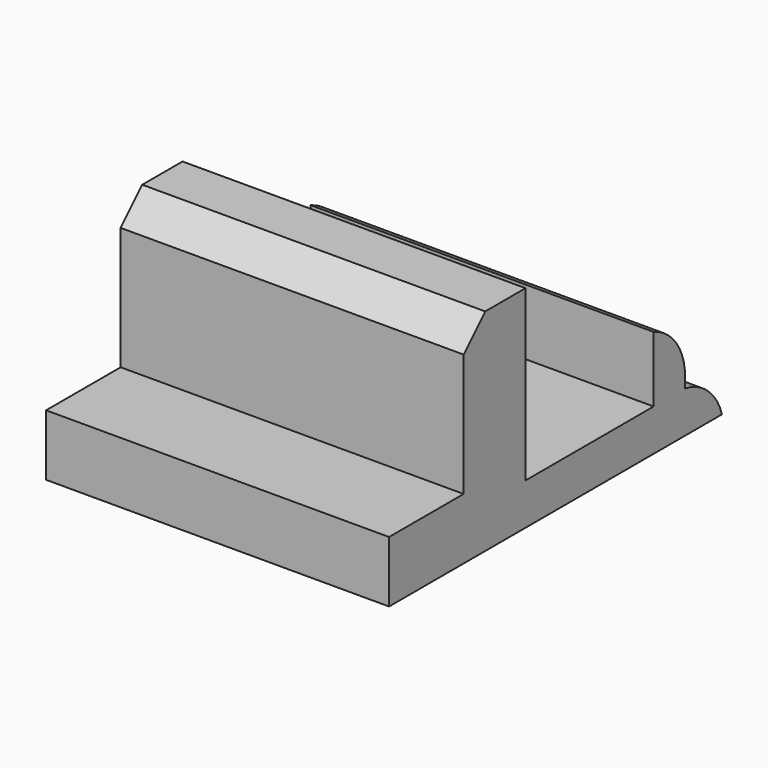
from build123d import *

# Parameters (mm, degrees)
F0_W        = 17.2521322966
F0_H        = 11.3339135423
F1_DEPTH    = 63.5
F2_T1_DEPTH = 116.9691747536
F2_T3_DEPTH = 114.7757874589
F3_SIZE     = 5


# Not quite as in the source:
# - a fillet or chamfer that OpenCascade refuses, or shapes differently, is made with other operations: its cross-section is extruded or revolved along the edge and cut away or added


with BuildPart() as f1:
    # F0 (on Right) → F1 (new body)
    with BuildSketch(Plane.YZ):
        Polygon((-28.8866702467, 39.0534885228), (-43.2048514485, 39.0534885228), (-43.2048514485, 11.3339135423), (-43.2048514485, 0), (16.9898695312, 0), (16.9898695312, 7.7048568055), (8.0409916118, 7.7048568055), (8.0409916118, 19.8725238442), (0.7627514424, 19.8725238442), (0.7627514424, 7.7155772597), (-28.8866702467, 7.7155772597), align=None)
        with Locations((-51.8309175968, 5.6669567712)):
            Rectangle(F0_W, F0_H)
    extrude(amount=F1_DEPTH)

    # F2: fillet of radius 10.8639610307 on 2 edges, made by hand

    # F2_s2 → F2_t1 (cut)
    with BuildSketch(Plane.YZ.offset(-26.7345873768)):
        with BuildLine():
            ThreePointArc((16.9898695312, -2.9889781452), (14.4575061135, 3.9831184184), (8.0409916118, 7.7048568055))
            Line((8.0409916118, 7.7048568055), (16.9898695312, 7.7048568055))
            Line((16.9898695312, 7.7048568055), (16.9898695312, -2.9889781452))
        make_face()
    extrude(amount=F2_T1_DEPTH, mode=Mode.SUBTRACT)

    # F2_s4 → F2_t3 (cut)
    with BuildSketch(Plane.YZ.offset(-25.6378937294)):
        with BuildLine():
            ThreePointArc((8.0409916118, 9.6173663525), (6.0365108418, 15.9050733102), (0.7627514424, 19.8725238442))
            Line((0.7627514424, 19.8725238442), (8.0409916118, 19.8725238442))
            Line((8.0409916118, 19.8725238442), (8.0409916118, 9.6173663525))
        make_face()
    extrude(amount=F2_T3_DEPTH, mode=Mode.SUBTRACT)

    # F3
    f3_edges = [f1.edges().sort_by_distance(p)[0] for p in [
        (31.75, -43.204851, 39.053489),
    ]]
    chamfer(f3_edges, length=F3_SIZE)


solid = f1.part
